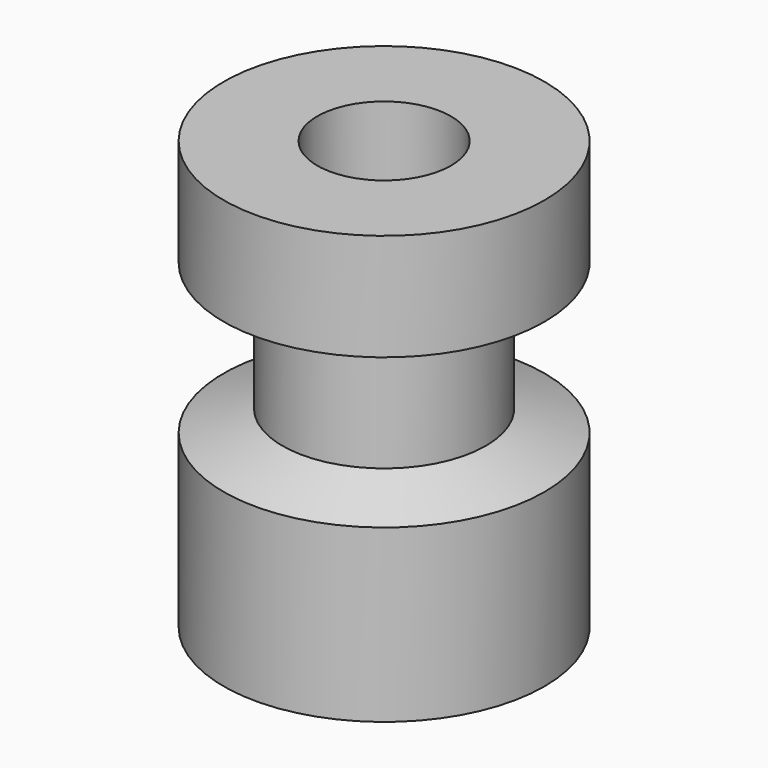
from build123d import *

# Parameters (mm, degrees)
F2_R     = 3.96875
F3_DEPTH = 25.401
F4_R     = 6.223
F4_R_2   = 3.96875
F5_DEPTH = 8.382


# Not quite as in the source:
# - a feature names something its author has since deleted; it is built from what else it names


with BuildPart() as f1:
    # F0 (on Front) → F1 (revolve)
    with BuildSketch(Plane.XZ):
        Polygon((0, 12.7), (0, 0), (0, -12.7), (9.525, -12.7), (9.525, -2.54), (6.0357036773, -1.27), (6.0357036773, 5.08), (9.525, 6.35), (9.525, 12.7), align=None)
    revolve(axis=Axis((0, 0, 2.3044683039), (0, 0, 1)))

    # F2 (on face) → F3 (cut, through all)
    with BuildSketch(Plane(origin=(0, 0, -12.7), x_dir=(1, 0, 0), z_dir=(0, 0, -1))):
        Circle(F2_R)
    extrude(amount=-F3_DEPTH, mode=Mode.SUBTRACT)

    # F4 (on face) → F5 (cut)
    with BuildSketch(Plane(origin=(0, 0, -12.7), x_dir=(1, 0, 0), z_dir=(0, 0, -1))):
        Circle(F4_R)
        Circle(F4_R_2, mode=Mode.SUBTRACT)
    extrude(amount=-F5_DEPTH, mode=Mode.SUBTRACT)


solid = f1.part
